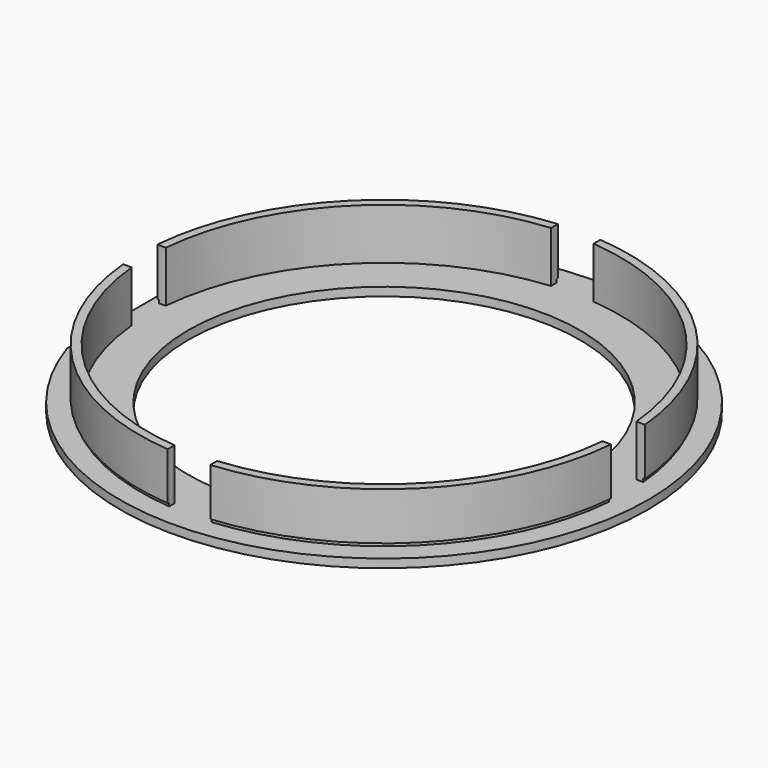
from build123d import *

# Parameters (mm, degrees)
F0_R          = 62
F1_DEPTH      = 2
F5_W          = 14.1073614359
F5_H          = 85.8036801219
F6_DEPTH      = 25
F4_R          = 55.5
F7_DEPTH      = 2
F8_R          = 57.1
F9_DEPTH      = 0.8
F10_R         = 57.5
F11_DEPTH     = 11.2
F12_R         = 46
F13_DEPTH     = 25
F14_R         = 55.5
F15_DEPTH     = 12
F16_W         = 10
F16_H         = 120
F17_DEPTH     = 12
F18_W         = 120
F18_H         = 10
F19_DEPTH     = 12
F20_TEXT_SIZE = 9.1257712079
F21_DEPTH     = 0.6


# Not quite as in the source:
# - a feature of the source that left no trace in its solid (it failed there, or was rolled back) is left out
# - a feature names something its author has since deleted; it is built from what else it names
# - Text() gives the source's letters only with a copy of the font that has no kerning and outlines rounded to 1/6400 em; it was checked with that copy


with BuildPart() as f1:
    # F0 (on Top) → F1 (new body)
    with BuildSketch(Plane.XY):
        Circle(F0_R)
    extrude(amount=F1_DEPTH)

    # F5 (on face) → F6 (cut)
    with BuildSketch(Plane.XY.offset(2)):
        with Locations((-65.8987760544, -2.3190192878)):
            Rectangle(F5_W, F5_H)
    extrude(amount=-F6_DEPTH, mode=Mode.SUBTRACT)

    # F4 (on face) + F1_face1 (on face) → F7 (cut)
    with BuildSketch(Plane.XY.offset(4)):
        Circle(F4_R)
    with BuildSketch(Plane(origin=(0.4137878861, 0, 0), x_dir=(1, 0, 0), z_dir=(0, 0, -1))):
        with BuildLine():
            ThreePointArc((-59.2588832226, -19.5257459485), (61.5862121139, 0), (-59.2588832226, 19.5257459485))
            Line((-59.2588832226, 19.5257459485), (-59.2588832226, -19.5257459485))
        make_face()
    extrude(amount=-F7_DEPTH, dir=(0, 0, 1), mode=Mode.SUBTRACT)

    # F8 (on face) → F9 (join)
    with BuildSketch(Plane.XY.offset(2)):
        Circle(F8_R)
    extrude(amount=F9_DEPTH)

    # F10 (on face) → F11 (join)
    with BuildSketch(Plane.XY.offset(2.8)):
        Circle(F10_R)
    extrude(amount=F11_DEPTH)

    # F12 (on face) → F13 (cut)
    with BuildSketch(Plane.XY.offset(14)):
        Circle(F12_R)
    extrude(amount=-F13_DEPTH, mode=Mode.SUBTRACT)

    # F14 (on face) → F15 (cut)
    with BuildSketch(Plane.XY.offset(14)):
        Circle(F14_R)
    extrude(amount=-F15_DEPTH, mode=Mode.SUBTRACT)

    # F16 (on face) → F17 (cut)
    with BuildSketch(Plane.XY.offset(14)):
        Rectangle(F16_W, F16_H)
    extrude(amount=-F17_DEPTH, mode=Mode.SUBTRACT)

    # F18 (on face) → F19 (cut)
    with BuildSketch(Plane.XY.offset(14)):
        Rectangle(F18_W, F18_H)
    extrude(amount=-F19_DEPTH, mode=Mode.SUBTRACT)

    # F20 (on face) → F21 (cut)
    with BuildSketch(Plane(origin=(0, 0, 0), x_dir=(1, 0, 0), z_dir=(0, 0, -1))):
        with Locations((-21.9340501353, 49.2791421711)):
            Text('MIYAUCHI', F20_TEXT_SIZE, font='Open Sans', font_style=FontStyle.BOLDITALIC, text_align=(TextAlign.LEFT, TextAlign.BOTTOM))
    extrude(amount=-F21_DEPTH, mode=Mode.SUBTRACT)


solid = f1.part
